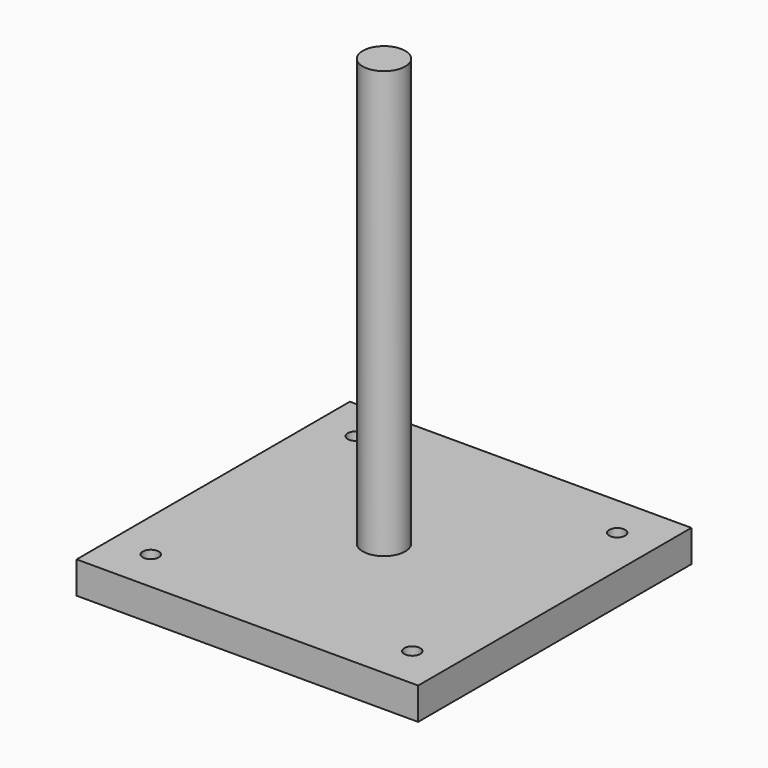
from build123d import *

# Parameters (mm, degrees)
F0_W     = 203.2
F0_H     = 203.2
F1_DEPTH = 19.05
F3_D     = 9.525
F4_R     = 12.6365
F5_DEPTH = 254


# Not quite as in the source:
# - a length typed as a fraction of an inch, garbled in the dataset ("3 / 203.2 mm" for 3/8 in), is restored


with BuildPart() as f1:
    # F0 (on Top) → F1 (new body)
    with BuildSketch(Plane.XY):
        Rectangle(F0_W, F0_H)
    extrude(amount=F1_DEPTH)

    # F3 (through all)
    with Locations(Plane.XY.offset(19.05)):
        with Locations((-77.7875, 76.2), (77.7875, 76.2), (-77.7875, -76.2), (77.7875, -76.2)):
            Hole(F3_D / 2)

    # F4 (on face) → F5 (join)
    with BuildSketch(Plane.XY.offset(19.05)):
        Circle(F4_R)
    extrude(amount=F5_DEPTH)


solid = f1.part
